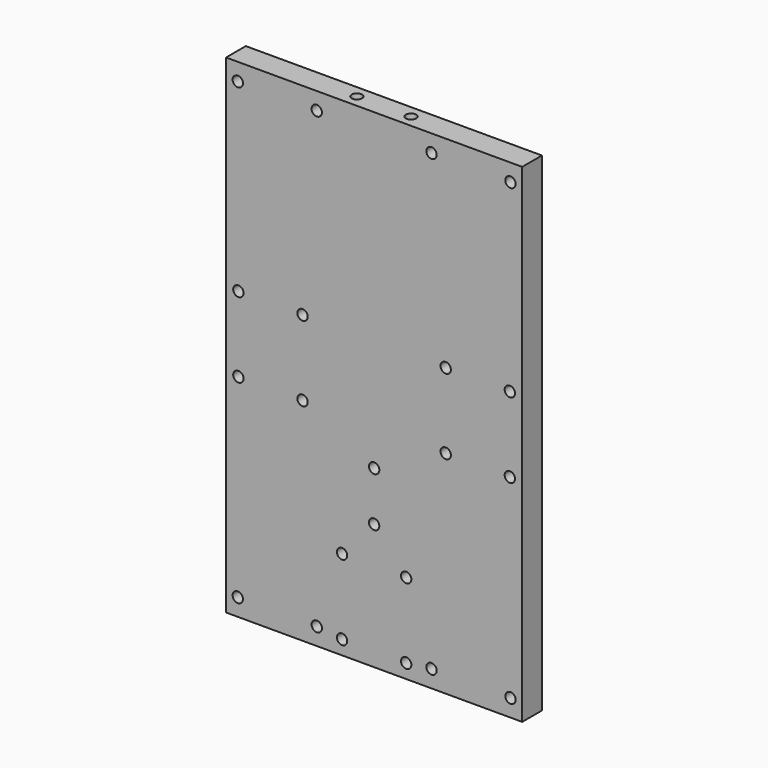
from build123d import *

# Parameters (mm, degrees)
F0_W     = 120
F0_H     = 122
F0_H_2   = 76
F1_DEPTH = 10
F3_D     = 4.2
F5_D     = 4.2
F7_D     = 4.2
F7_DEPTH = 12.4
F7_TIP   = 1.2618073


# Not quite as in the source:
# - a feature names something its author has since deleted; it is built from what else it names


with BuildPart() as f1:
    # F0 (on Front) → F1 (new body)
    with BuildSketch(Plane.XZ):
        Rectangle(F0_W, F0_H)
        with Locations((0, 99)):
            Rectangle(F0_W, F0_H_2)
    extrude(amount=F1_DEPTH)

    # F3 (through all)
    with Locations(Plane(origin=(0, 0, 0), x_dir=(-1, 0, 0), z_dir=(0, 1, 0))):
        with Locations((-55, 55.25), (-29, 55.25), (-29, 24.75), (-55, 24.75), (29, 55.25), (55, 55.25), (55, 24.75), (29, 24.75), (-13, -24.75), (13, -24.75), (13, -55.25), (-13, -55.25), (0, 10), (0, -10)):
            Hole(F3_D / 2)

    # F5 (through all)
    with Locations(Plane(origin=(0, 0, 0), x_dir=(-1, 0, 0), z_dir=(0, 1, 0))):
        with Locations((-55.25, 130), (-23.25, 130), (23.25, 130), (55.25, 130), (-55.25, -54), (-23.25, -54), (23.25, -54), (55.25, -54)):
            Hole(F5_D / 2)

    # F7
    with Locations(Plane.XY.offset(137)):
        with Locations((11, -5), (-11, -5)):
            Hole(F7_D / 2, depth=F7_DEPTH)
            with Locations((0, 0, -(F7_DEPTH + F7_TIP / 2))):  # 118° drill point
                Cone(0, F7_D / 2, F7_TIP, mode=Mode.SUBTRACT)


solid = f1.part
